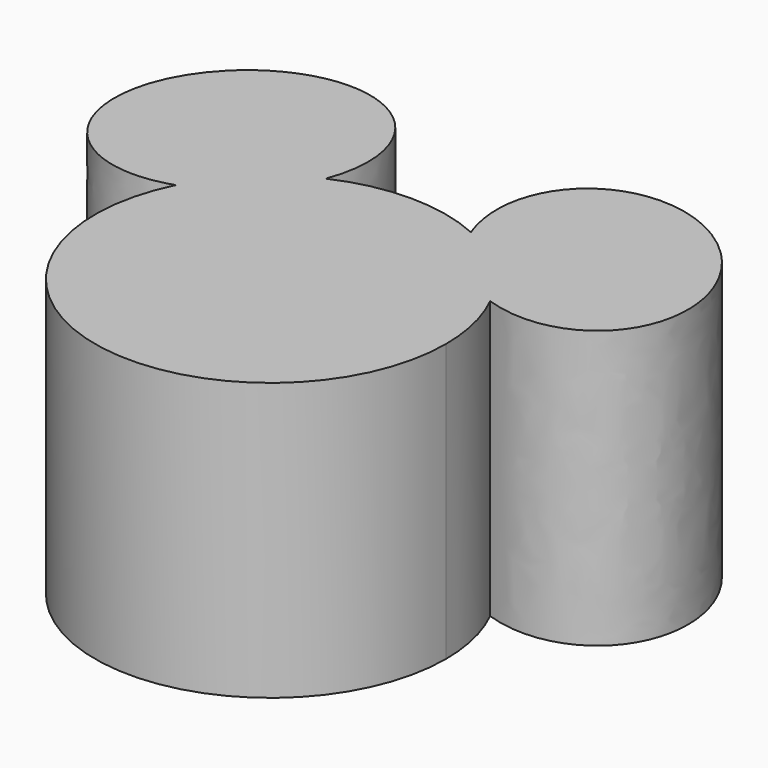
from build123d import *

# Parameters (mm, degrees)
F1_DEPTH = 25.4


with BuildPart() as f1:
    # F0 (on Top) → F1 (new body)
    with BuildSketch(Plane.XY):
        with BuildLine():
            ThreePointArc((-14.3874178664, 24.3026331135), (-3.6778055907, 1.497966924), (16.0707555221, 17.1422287822))
            ThreePointArc((16.0707555221, 17.1422287822), (15.6442618582, 20.8200343728), (14.3874178664, 24.3026331135))
            add(Edge.make_bspline(
                [(6.6488676301, 31.7730777763), (8.7871476467, 26.2175508691), (14.3874178664, 24.3026331135)],
                knots=[1.0830446402, 1.0830446402, 1.0830446402, 2.100651681, 2.100651681, 2.100651681], degree=2, weights=[1, 0.8733279769, 1]))
            ThreePointArc((6.6488676301, 31.7730777763), (0, 33.2129843043), (-6.6488676301, 31.7730777763))
            add(Edge.make_bspline(
                [(-14.3874178664, 24.3026331135), (-8.7871476467, 26.2175508691), (-6.6488676301, 31.7730777763)],
                knots=[1.0409409725, 1.0409409725, 1.0409409725, 2.0585480134, 2.0585480134, 2.0585480134], degree=2, weights=[1, 0.8733279769, 1]))
        make_face()
        with BuildLine():
            add(Edge.make_bspline(
                [(6.6488676301, 31.7730777763), (8.7871476467, 26.2175508691), (14.3874178664, 24.3026331135)],
                knots=[1.0830446402, 1.0830446402, 1.0830446402, 2.100651681, 2.100651681, 2.100651681], degree=2, weights=[1, 0.8733279769, 1]))
            ThreePointArc((14.3874178664, 24.3026331135), (11.1616850313, 28.7044937122), (6.6488676301, 31.7730777763))
        make_face()
        with BuildLine():
            ThreePointArc((6.6488676301, 31.7730777763), (11.1616850313, 28.7044937122), (14.3874178664, 24.3026331135))
            add(Edge.make_bspline(
                [(14.3874178664, 24.3026331135), (51.3942103362, 11.6487858527), (22.6181104936, 40.4248756132)],
                knots=[2.100651681, 2.100651681, 2.100651681, 4.7123889804, 4.7123889804, 4.7123889804], degree=2, weights=[1, 0.2618394692, 1]))
            add(Edge.make_bspline(
                [(22.6181104936, 40.4248756132), (16.5155810704, 46.5274028982), (10.0839719096, 43.0428931628), (3.6523627487, 39.5583834273), (6.6488676301, 31.7730777763)],
                knots=[4.7123889804, 4.7123889804, 4.7123889804, 6.0393094639, 6.0393094639, 7.3662299474, 7.3662299474, 7.3662299474], degree=2, weights=[1, 0.7878659738, 1, 0.7878659738, 1]))
        make_face()
        with BuildLine():
            add(Edge.make_bspline(
                [(-22.6181104936, 40.4248756132), (-51.3942103362, 11.6487858527), (-14.3874178664, 24.3026331135)],
                knots=[4.7123889804, 4.7123889804, 4.7123889804, 7.3241262797, 7.3241262797, 7.3241262797], degree=2, weights=[1, 0.2618394692, 1]))
            ThreePointArc((-14.3874178664, 24.3026331135), (-11.1616850313, 28.7044937122), (-6.6488676301, 31.7730777763))
            add(Edge.make_bspline(
                [(-6.6488676301, 31.7730777763), (-3.6523627487, 39.5583834273), (-10.0839719096, 43.0428931628), (-16.5155810704, 46.5274028982), (-22.6181104936, 40.4248756132)],
                knots=[2.0585480134, 2.0585480134, 2.0585480134, 3.3854684969, 3.3854684969, 4.7123889804, 4.7123889804, 4.7123889804], degree=2, weights=[1, 0.7878659738, 1, 0.7878659738, 1]))
        make_face()
        with BuildLine():
            ThreePointArc((-6.6488676301, 31.7730777763), (-11.1616850313, 28.7044937122), (-14.3874178664, 24.3026331135))
            add(Edge.make_bspline(
                [(-14.3874178664, 24.3026331135), (-8.7871476467, 26.2175508691), (-6.6488676301, 31.7730777763)],
                knots=[1.0409409725, 1.0409409725, 1.0409409725, 2.0585480134, 2.0585480134, 2.0585480134], degree=2, weights=[1, 0.8733279769, 1]))
        make_face()
    extrude(amount=F1_DEPTH)


solid = f1.part
